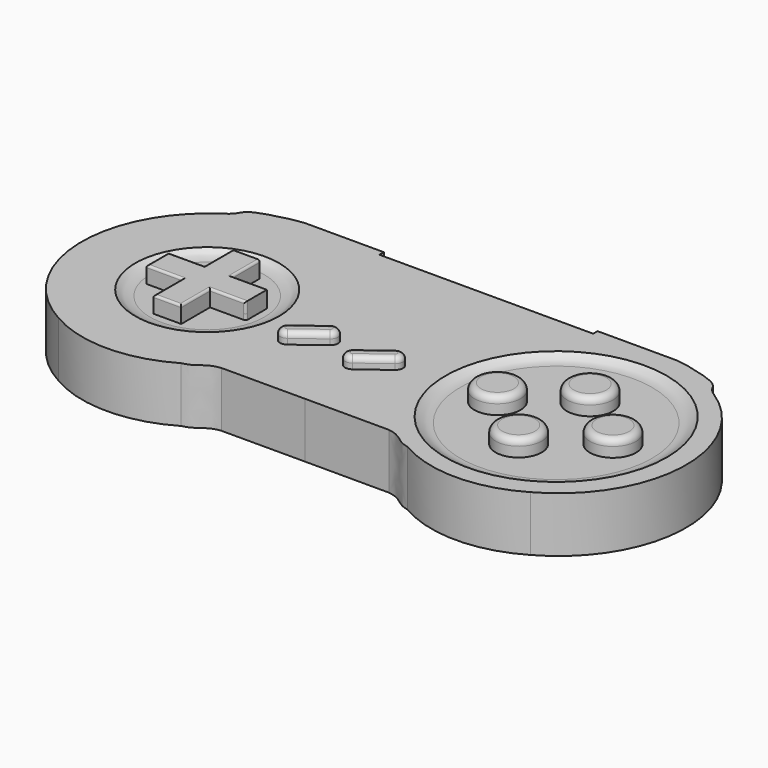
from build123d import *

# Parameters (mm, degrees)
F1_DEPTH     = 12.7
F2_R         = 5.2959
F3_DEPTH     = 2.54
F4_R         = 0.508
F5_R         = 1.27
F6_R         = 1.524
F7_R         = 16.51
F7_R_2       = 25.4
F7_R_3       = 5.2959
F8_DEPTH     = 1.27
F9_T1_DEPTH  = 12.7
F10_T1_DEPTH = 12.7


# Not quite as in the source:
# - a fillet or chamfer that OpenCascade refuses, or shapes differently, is made with other operations: its cross-section is extruded or revolved along the edge and cut away or added


with BuildPart() as f1:
    # F0 (on Top) → F1 (new body)
    with BuildSketch(Plane.XY):
        with BuildLine():
            Line((0, -25.6294570863), (0, 0))
            Line((0, 0), (0, 26.3838227838))
            Line((0, 26.3838227838), (-24.5490502566, 26.3838227838))
            Line((-24.5490502566, 26.3838227838), (-24.5490502566, 27.6538227838))
            Line((-24.5490502566, 27.6538227838), (-42.7472442389, 27.6538227838))
            add(Edge.make_bspline(
                [(-42.7472442389, 27.6538227838), (-43.4760030996, 27.5730225568), (-45.4153628334, 27.3579984724), (-52.8813355612, 25.3954780063), (-53.8498209002, 24.1242184105), (-54.1770942509, 23.6946307123)],
                knots=[0, 0, 0, 0, 0.2849777741, 0.7583776333, 1, 1, 1, 1], degree=3))
            Line((-54.1770942509, 23.6946307123), (-54.1770942509, 22.698847577))
            ThreePointArc((-54.1770942509, 22.698847577), (-69.3989631751, -3.0011655763), (-54.1770942509, -28.7011787295))
            ThreePointArc((-54.1770942509, -28.7011787295), (-40.0796784088, -32.5237378873), (-25.9822625667, -28.7011787295))
            add(Edge.make_bspline(
                [(-25.9822625667, -28.7011787295), (-25.4343945091, -28.56295557), (-24.3230926927, -28.2825821367), (-22.9565361011, -27.1750055362), (-21.0017610227, -25.9362543342), (-19.795647402, -25.7391331905), (-19.230728969, -25.6468057632)],
                knots=[0, 0, 0, 0, 0.2363797592, 0.4794753994, 0.7561971471, 1, 1, 1, 1], degree=3))
            Line((-19.230728969, -25.6468057632), (0, -25.6294570863))
        make_face()
        with BuildLine():
            Line((0, 26.3838227838), (0, 0))
            Line((0, 0), (0, -25.6294570863))
            Line((0, -25.6294570863), (19.230728969, -25.6468057632))
            add(Edge.make_bspline(
                [(25.9822625667, -28.7011787295), (25.4343945091, -28.56295557), (24.3230926927, -28.2825821367), (22.9565361011, -27.1750055362), (21.0017610227, -25.9362543342), (19.795647402, -25.7391331905), (19.230728969, -25.6468057632)],
                knots=[0, 0, 0, 0, 0.2363797592, 0.4794753994, 0.7561971471, 1, 1, 1, 1], degree=3))
            ThreePointArc((25.9822625667, -28.7011787295), (40.0796784088, -32.5237378873), (54.1770942509, -28.7011787295))
            ThreePointArc((54.1770942509, -28.7011787295), (69.3989631751, -3.0011655763), (54.1770942509, 22.698847577))
            Line((54.1770942509, 22.698847577), (54.1770942509, 23.6946307123))
            add(Edge.make_bspline(
                [(42.7472442389, 27.6538227838), (43.4760030996, 27.5730225568), (45.4153628334, 27.3579984724), (52.8813355612, 25.3954780063), (53.8498209002, 24.1242184105), (54.1770942509, 23.6946307123)],
                knots=[0, 0, 0, 0, 0.2849777741, 0.7583776333, 1, 1, 1, 1], degree=3))
            Line((42.7472442389, 27.6538227838), (24.5490502566, 27.6538227838))
            Line((24.5490502566, 27.6538227838), (24.5490502566, 26.3838227838))
            Line((24.5490502566, 26.3838227838), (0, 26.3838227838))
        make_face()
    extrude(amount=F1_DEPTH)

    # F2 (on face) → F3 (join)
    with BuildSketch(Plane.XY.offset(12.7)):
        Polygon((-51.6182854772, -0.3126390842), (-51.6182854772, -3.4876390842), (-51.6182854772, -6.6626390842), (-43.3632854772, -6.6626390842), (-43.3632854772, -14.9176390842), (-40.1882854772, -14.9176390842), (-37.0132854772, -14.9176390842), (-37.0132854772, -6.6626390842), (-28.7582854772, -6.6626390842), (-28.7582854772, -3.4876390842), (-28.7582854772, -0.3126390842), (-37.0132854772, -0.3126390842), (-37.0132854772, 7.9423609158), (-40.1882854772, 7.9423609158), (-43.3632854772, 7.9423609158), (-43.3632854772, -0.3126390842), align=None)
        with BuildLine():
            Line((-11.6528549959, -3.7563646925), (-17.7488548827, -8.3283648434))
            ThreePointArc((-17.7488548827, -8.3283648434), (-18.1044548211, -10.8175648522), (-15.6152548123, -11.1731647906))
            Line((-15.6152548123, -11.1731647906), (-9.5192549254, -6.6011646397))
            ThreePointArc((-9.5192549254, -6.6011646397), (-9.1636549871, -4.1119646309), (-11.6528549959, -3.7563646925))
        make_face()
        with BuildLine():
            Line((3.4466944985, -3.9755433972), (-2.6493053883, -8.547543548))
            ThreePointArc((-2.6493053883, -8.547543548), (-3.0049053267, -11.0367435568), (-0.5157053179, -11.3923434952))
            Line((-0.5157053179, -11.3923434952), (5.5802945689, -6.8203433443))
            ThreePointArc((5.5802945689, -6.8203433443), (5.9358945073, -4.3311433355), (3.4466944985, -3.9755433972))
        make_face()
        with Locations((26.0627494857, -2.9921420355)):
            Circle(F2_R)
        with Locations((39.3263548613, 7.014032919)):
            Circle(F2_R)
        with Locations((52.5939278305, -2.9921420355)):
            Circle(F2_R)
        with Locations((39.3263548613, -13.4836789221)):
            Circle(F2_R)
    extrude(amount=F3_DEPTH)

    # F4
    f4_edges = [f1.edges().sort_by_distance(p)[0] for p in [
        (-43.363285, 7.942361, 13.97),
        (-40.188285, 7.942361, 15.24),
        (-37.013285, 7.942361, 13.97),
        (-37.013285, 3.814861, 15.24),
        (-32.885785, -0.312639, 15.24),
        (-28.758285, -0.312639, 13.97),
        (-28.758285, -6.662639, 13.97),
        (-32.885785, -6.662639, 15.24),
        (-47.490785, -6.662639, 15.24),
        (-47.490785, -0.312639, 15.24),
        (-43.363285, 3.814861, 15.24),
        (-51.618285, -3.487639, 15.24),
        (-40.188285, -14.917639, 15.24),
        (-43.363285, -10.790139, 15.24),
        (-37.013285, -10.790139, 15.24),
    ]]
    fillet(f4_edges, radius=F4_R)

    # F5
    f5_edges = [f1.edges().sort_by_distance(p)[0] for p in [
        (-14.700855, -6.042365, 15.24),
        (0.398695, -6.261543, 15.24),
        (-18.104455, -10.817565, 15.24),
        (-12.567255, -8.887165, 15.24),
        (-9.163655, -4.111965, 15.24),
        (5.935895, -4.331143, 15.24),
        (-3.004905, -11.036744, 15.24),
        (2.532295, -9.106343, 15.24),
    ]]
    fillet(f5_edges, radius=F5_R)

    # F6
    f6_edges = [f1.edges().sort_by_distance(p)[0] for p in [
        (20.766849, -2.992142, 15.24),
        (47.298028, -2.992142, 15.24),
        (34.030455, 7.014033, 15.24),
        (34.030455, -13.483679, 15.24),
    ]]
    fillet(f6_edges, radius=F6_R)

    # F7 (on face) → F8 (cut)
    with BuildSketch(Plane.XY.offset(12.7)):
        with Locations((-40.1882854772, -3.4876391292)):
            Circle(F7_R)
        with BuildLine():
            ThreePointArc((-28.7582854772, -6.1546390842), (-28.9070752323, -6.513849329), (-29.2662854772, -6.6626390842))
            Line((-29.2662854772, -6.6626390842), (-37.0132854772, -6.6626390842))
            Line((-37.0132854772, -6.6626390842), (-37.0132854772, -14.9176390842))
            Line((-37.0132854772, -14.9176390842), (-43.3632854772, -14.9176390842))
            Line((-43.3632854772, -14.9176390842), (-43.3632854772, -6.6626390842))
            Line((-43.3632854772, -6.6626390842), (-51.6182854772, -6.6626390842))
            Line((-51.6182854772, -6.6626390842), (-51.6182854772, -0.3126390842))
            Line((-51.6182854772, -0.3126390842), (-43.3632854772, -0.3126390842))
            Line((-43.3632854772, -0.3126390842), (-43.3632854772, 7.4343609158))
            ThreePointArc((-43.3632854772, 7.4343609158), (-43.214495722, 7.7935711607), (-42.8552854772, 7.9423609158))
            Line((-42.8552854772, 7.9423609158), (-37.5212854772, 7.9423609158))
            ThreePointArc((-37.5212854772, 7.9423609158), (-37.1620752323, 7.7935711607), (-37.0132854772, 7.4343609158))
            Line((-37.0132854772, 7.4343609158), (-37.0132854772, -0.3126390842))
            Line((-37.0132854772, -0.3126390842), (-29.2662854772, -0.3126390842))
            ThreePointArc((-29.2662854772, -0.3126390842), (-28.9070752323, -0.4614288393), (-28.7582854772, -0.8206390842))
            Line((-28.7582854772, -0.8206390842), (-28.7582854772, -6.1546390842))
        make_face(mode=Mode.SUBTRACT)
        with Locations((39.4583567977, -2.8860671446)):
            Circle(F7_R_2)
        with Locations((26.0627494857, -2.9921420355)):
            Circle(F7_R_3, mode=Mode.SUBTRACT)
        with Locations((39.3263548613, -13.4836789221)):
            Circle(F7_R_3, mode=Mode.SUBTRACT)
        with Locations((52.5939278305, -2.9921420355)):
            Circle(F7_R_3, mode=Mode.SUBTRACT)
        with Locations((39.3263548613, 7.014032919)):
            Circle(F7_R_3, mode=Mode.SUBTRACT)
    extrude(amount=-F8_DEPTH, mode=Mode.SUBTRACT)

    # F9: fillet of radius 5.08 on 1 edges, made by hand

    # F9_s2 → F9_t1 (join)
    with BuildSketch(Plane.XY):
        with BuildLine():
            ThreePointArc((-56.0076348906, 21.607272627), (-54.9470006237, 22.52347253), (-54.1770942509, 23.6946307123))
            Line((-54.1770942509, 23.6946307123), (-54.0853087769, 23.6510648225))
            ThreePointArc((-54.0853087769, 23.6510648225), (-54.0754942509, 23.1967391446), (-54.0754942509, 22.698847577))
            Line((-54.0754942509, 22.698847577), (-54.1282657465, 22.6097502305))
            ThreePointArc((-54.1282657465, 22.6097502305), (-55.0502548962, 22.0824433564), (-55.9524602294, 21.5219595755))
            Line((-55.9524602294, 21.5219595755), (-56.0076348906, 21.607272627))
        make_face()
    extrude(amount=F9_T1_DEPTH)

    # F10: fillet of radius 5.08 on 1 edges, made by hand

    # F10_s2 → F10_t1 (join)
    with BuildSketch(Plane.XY):
        with BuildLine():
            ThreePointArc((54.1770942509, 23.6946307123), (54.9470006237, 22.52347253), (56.0076348906, 21.607272627))
            Line((56.0076348906, 21.607272627), (55.9524602294, 21.5219595755))
            ThreePointArc((55.9524602294, 21.5219595755), (55.0502548962, 22.0824433564), (54.1282657465, 22.6097502305))
            Line((54.1282657465, 22.6097502305), (54.0754942509, 22.698847577))
            ThreePointArc((54.0754942509, 22.698847577), (54.0754942509, 23.1967391446), (54.0853087769, 23.6510648225))
            Line((54.0853087769, 23.6510648225), (54.1770942509, 23.6946307123))
        make_face()
    extrude(amount=F10_T1_DEPTH)

    # F11: fillet of radius 5.08 on 2 edges, made by hand

    # F11_s1 → F11_t2 (revolve)
    with BuildSketch(Plane.XZ.offset(2.8860671446)):
        with BuildLine():
            ThreePointArc((61.4982526326, 11.43), (63.2943038569, 11.7580951188), (64.8583567977, 12.7))
            Line((64.8583567977, 12.7), (64.8583567977, 11.43))
            Line((64.8583567977, 11.43), (61.4982526326, 11.43))
        make_face()
    revolve(axis=Axis((39.4583567977, -2.8860671446, 11.43), (0, 0, 1)))

    # F11_s3 → F11_t4 (revolve)
    with BuildSketch(Plane.XZ.offset(3.4876391292)):
        with BuildLine():
            ThreePointArc((-23.6782854772, 12.7), (-25.242338418, 11.7580951188), (-27.0383896422, 11.43))
            Line((-27.0383896422, 11.43), (-23.6782854772, 11.43))
            Line((-23.6782854772, 11.43), (-23.6782854772, 12.7))
        make_face()
    revolve(axis=Axis((-40.1882854772, -3.4876391292, 11.43), (0, 0, 1)))


solid = f1.part
